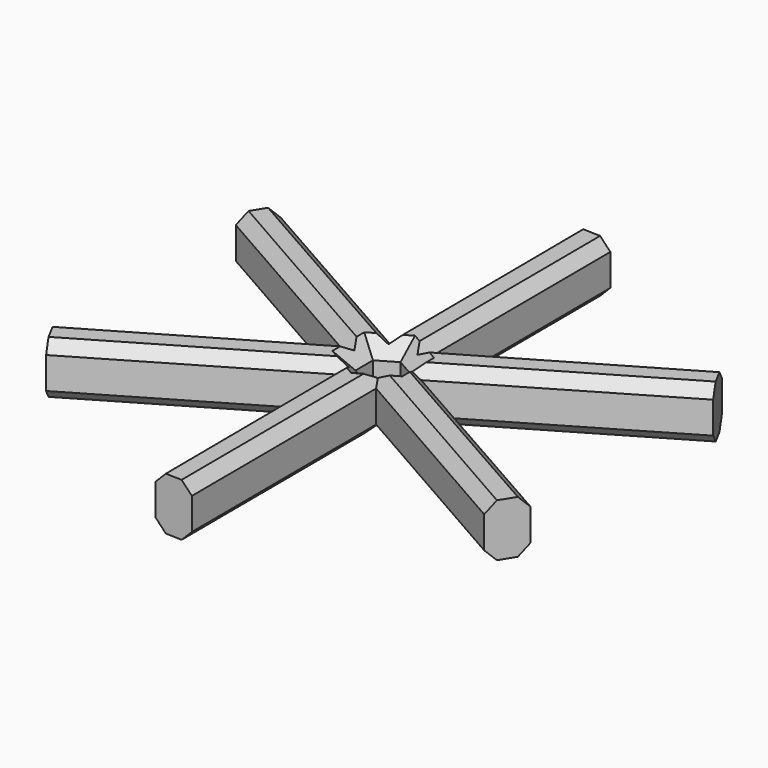
from build123d import *

# Parameters (mm, degrees)
F1_DEPTH      = 12.7
F2_SIZE       = 3.81
F3_T4_DEPTH   = 68.8298051047
F3_T9_DEPTH   = 68.1650882882
F3_T14_DEPTH  = 68.5414410237
F3_T19_DEPTH  = 68.5009740433
F3_T24_DEPTH  = 68.8298051047
F3_T29_DEPTH  = 68.1650882882
F3_T34_DEPTH  = 68.5414410237
F3_T39_DEPTH  = 68.5009740433
F3_T44_DEPTH  = 68.8298051047
F3_T49_DEPTH  = 68.1650882882
F3_T54_DEPTH  = 68.5414410237
F3_T59_DEPTH  = 68.5009740433
F3_T64_DEPTH  = 68.8298051047
F3_T69_DEPTH  = 68.1650882882
F3_T74_DEPTH  = 68.5414410237
F3_T79_DEPTH  = 68.5009740433
F3_T84_DEPTH  = 68.8298051047
F3_T89_DEPTH  = 68.1650882882
F3_T94_DEPTH  = 68.5414410237
F3_T99_DEPTH  = 68.5009740433
F3_T104_DEPTH = 68.8298051047
F3_T109_DEPTH = 68.1650882882
F3_T114_DEPTH = 68.5414410237
F3_T119_DEPTH = 68.5009740433
F3_T125_DEPTH = 68.8298051047
F3_T130_DEPTH = 68.1650882882
F3_T138_DEPTH = 68.5414410237
F3_T143_DEPTH = 68.5009740433
F3_T151_DEPTH = 68.8298051047
F3_T156_DEPTH = 68.1650882882
F3_T164_DEPTH = 68.5414410237
F3_T169_DEPTH = 68.5009740433
F3_T177_DEPTH = 68.8298051047
F3_T182_DEPTH = 68.1650882882
F3_T190_DEPTH = 68.5414410237
F3_T195_DEPTH = 68.5009740433
F3_T203_DEPTH = 68.8298051047
F3_T208_DEPTH = 68.1650882882
F3_T216_DEPTH = 68.5414410237
F3_T221_DEPTH = 68.5009740433
F3_T229_DEPTH = 68.8298051047
F3_T234_DEPTH = 68.1650882882
F3_T242_DEPTH = 68.5414410237
F3_T247_DEPTH = 68.5009740433
F3_T255_DEPTH = 68.8298051047
F3_T260_DEPTH = 68.1650882882
F3_T268_DEPTH = 68.5414410237
F3_T273_DEPTH = 68.5009740433


# Not quite as in the source:
# - a fillet or chamfer that OpenCascade refuses, or shapes differently, is made with other operations: its cross-section is extruded or revolved along the edge and cut away or added


with BuildPart() as f1:
    # F0 (on Top) → F1 (new body)
    with BuildSketch(Plane.XY):
        Polygon((4.2501981695, 63.0203421564), (-4.9943139693, 63.317529994), (-4.6016708631, 7.8416280415), (-0.0452432376, 5.2537971809), (4.5209166317, 7.9200684896), align=None)
        Polygon((-0.0452432376, 5.2537971809), (-4.6016708631, 7.8416280415), (-4.5646768909, 2.6148102364), align=None)
        Polygon((-4.5646768909, 2.6148102364), (-4.6016708631, 7.8416280415), (-52.8063450462, 35.2195551654), (-57.5503224335, 27.6004082668), (-9.1194388276, -0.0448055934), align=None)
        Polygon((-4.5273002062, -2.6660803836), (-4.5646768909, 2.6148102364), (-9.1194388276, -0.0448055934), align=None)
        Polygon((4.5209166317, 7.9200684896), (-0.0452432376, 5.2537971809), (4.5468305363, 2.6457210293), align=None)
        Polygon((52.6778159307, 36.03983709), (4.5209166317, 7.9200684896), (4.5468305363, 2.6457210293), (9.0918845225, 0.0643498466), (56.9042020064, 28.1218587083), align=None)
        Polygon((0.0178463546, -5.2605312658), (-4.5273002062, -2.6660803836), (-4.4902136594, -7.9059778881), align=None)
        Polygon((-4.4902136594, -7.9059778881), (-4.5273002062, -2.6660803836), (-9.1194388276, -0.0448055934), (-56.7023163474, -27.8293914923), (-52.3374324951, -35.9839677689), align=None)
        Polygon((9.0918845225, 0.0643498466), (4.5468305363, 2.6457210293), (4.5725434438, -2.5877167973), align=None)
        Polygon((0.0178463546, -5.2605312658), (-4.4902136594, -7.9059778881), (-4.0978569602, -63.3414138737), (4.8725065029, -63.6402453568), (4.5985221959, -7.8752628962), align=None)
        Polygon((4.5725434438, -2.5877167973), (0.0178463546, -5.2605312658), (4.5985221959, -7.8752628962), align=None)
        Polygon((9.0918845225, 0.0643498466), (4.5725434438, -2.5877167973), (4.5985221959, -7.8752628962), (52.4521181779, -35.1909506641), (57.3317464644, -27.3335622251), align=None)
    extrude(amount=F1_DEPTH)

    # F2
    f2_edges = [f1.edges().sort_by_distance(p)[0] for p in [
        (2.295195, -3.924124, 12.7),
        (-2.254727, -3.963306, 12.7),
        (-4.545989, -0.025635, 12.7),
        (-2.30496, 3.934304, 12.7),
        (2.250794, 3.949759, 12.7),
        (4.559687, 0.029002, 12.7),
        (-2.254727, -3.963306, 0),
        (2.295195, -3.924124, 0),
        (4.559687, 0.029002, 0),
        (2.250794, 3.949759, 0),
        (-2.30496, 3.934304, 0),
        (-4.545989, -0.025635, 0),
    ]]
    chamfer(f2_edges, length=F2_SIZE)

    # F3: chamfer of 2.54 on 24 edges, made by hand


with BuildPart() as f3_tool2:
    # F3_s3 → F3_t4 (new body)
    with BuildSketch(Plane(origin=(0.3448800676, -70.1946441039, 0), x_dir=(0, 0, 1), z_dir=(-0.004913137, 0.9999879305, 0))):
        Polygon((0, 2.0197744481), (2.54, 4.5597744481), (0, 4.5597744481), align=None)
    extrude(amount=F3_T4_DEPTH)

    split(bisect_by=Plane(origin=(-2.2604583159, -3.9600342448, 0), x_dir=(0, 0, 1), z_dir=(-0.4957390638, -0.8684715198, 0)), keep=Keep.TOP)


with BuildPart() as f1_1:
    add(f1.part)

    # F3_t1: cut F3_tool2
    add(f3_tool2.part, mode=Mode.SUBTRACT)


with BuildPart() as f3_tool7:
    # F3_s8 → F3_t9 (new body)
    with BuildSketch(Plane(origin=(1.186059592, -0.6770240109, 0), x_dir=(0, 0, 1), z_dir=(0.8684715198, -0.4957390638, 0))):
        Polygon((0, 2.0197744481), (2.54, 4.5597744481), (0, 4.5597744481), align=None)
    extrude(amount=F3_T9_DEPTH)

    split(bisect_by=Plane(origin=(4.5597194138, 0.0224027967, 0), x_dir=(0, 0, 1), z_dir=(0.9999879305, 0.004913137, 0)), keep=Keep.TOP)


with BuildPart() as f1_2:
    add(f1_1.part)

    # F3_t6: cut F3_tool7
    add(f3_tool7.part, mode=Mode.SUBTRACT)


with BuildPart() as f3_tool12:
    # F3_s13 → F3_t14 (new body)
    with BuildSketch(Plane(origin=(60.7665561884, -34.5124694876, 0), x_dir=(0, 0, 1), z_dir=(-0.8695424864, 0.4938581419, 0))):
        Polygon((0, 2.0060561225), (2.54, 4.5460561225), (0, 4.5460561225), align=None)
    extrude(amount=F3_T14_DEPTH)

    split(bisect_by=Plane(origin=(2.3008354316, -3.9208140208, 0), x_dir=(0, 0, 1), z_dir=(0.5061168119, -0.86246494, 0)), keep=Keep.TOP)


with BuildPart() as f1_3:
    add(f1_2.part)

    # F3_t11: cut F3_tool12
    add(f3_tool12.part, mode=Mode.SUBTRACT)


with BuildPart() as f3_tool17:
    # F3_s18 → F3_t19 (new body)
    with BuildSketch(Plane(origin=(1.1573635998, 0.6791709996, 0), x_dir=(0, 0, 1), z_dir=(0.86246494, 0.5061168119, 0))):
        Polygon((0, 2.0060561225), (2.54, 4.5460561225), (0, 4.5460561225), align=None)
    extrude(amount=F3_T19_DEPTH)

    split(bisect_by=Plane(origin=(2.2451068297, 3.952988944, 0), x_dir=(0, 0, 1), z_dir=(0.4938581419, 0.8695424864, 0)), keep=Keep.TOP)


with BuildPart() as f1_4:
    add(f1_3.part)

    # F3_t16: cut F3_tool17
    add(f3_tool17.part, mode=Mode.SUBTRACT)


with BuildPart() as f3_tool22:
    # F3_s23 → F3_t24 (new body)
    with BuildSketch(Plane(origin=(60.6179049697, 35.3959969517, 0), x_dir=(0, 0, 1), z_dir=(-0.8635583828, -0.5042488667, 0))):
        Polygon((0, 2.0197744481), (2.54, 4.5597744481), (0, 4.5597744481), align=None)
    extrude(amount=F3_T24_DEPTH)

    split(bisect_by=Plane(origin=(4.5597194138, 0.0224027967, 0), x_dir=(0, 0, 1), z_dir=(0.9999879305, 0.004913137, 0)), keep=Keep.TOP)


with BuildPart() as f1_5:
    add(f1_4.part)

    # F3_t21: cut F3_tool22
    add(f3_tool22.part, mode=Mode.SUBTRACT)


with BuildPart() as f3_tool27:
    # F3_s28 → F3_t29 (new body)
    with BuildSketch(Plane(origin=(-0.0067098036, 1.3656697426, 0), x_dir=(0, 0, 1), z_dir=(-0.004913137, 0.9999879305, 0))):
        Polygon((0, 2.0197744481), (2.54, 4.5597744481), (0, 4.5597744481), align=None)
    extrude(amount=F3_T29_DEPTH)

    split(bisect_by=Plane(origin=(-2.2992610979, 3.9376314481, 0), x_dir=(0, 0, 1), z_dir=(-0.5042488667, 0.8635583828, 0)), keep=Keep.TOP)


with BuildPart() as f1_6:
    add(f1_5.part)

    # F3_t26: cut F3_tool27
    add(f3_tool27.part, mode=Mode.SUBTRACT)


with BuildPart() as f3_tool32:
    # F3_s33 → F3_t34 (new body)
    with BuildSketch(Plane(origin=(-0.4946027707, 69.8816161035, 0), x_dir=(0, 0, 1), z_dir=(0.0070775464, -0.9999749539, 0))):
        Polygon((0, 2.0060561225), (2.54, 4.5460561225), (0, 4.5460561225), align=None)
    extrude(amount=F3_T34_DEPTH)

    split(bisect_by=Plane(origin=(2.2451068297, 3.952988944, 0), x_dir=(0, 0, 1), z_dir=(0.4938581419, 0.8695424864, 0)), keep=Keep.TOP)


with BuildPart() as f1_7:
    add(f1_6.part)

    # F3_t31: cut F3_tool32
    add(f3_tool32.part, mode=Mode.SUBTRACT)


with BuildPart() as f3_tool37:
    # F3_s38 → F3_t39 (new body)
    with BuildSketch(Plane(origin=(-1.1668611391, 0.6627207791, 0), x_dir=(0, 0, 1), z_dir=(-0.8695424864, 0.4938581419, 0))):
        Polygon((0, 2.0060561225), (2.54, 4.5460561225), (0, 4.5460561225), align=None)
    extrude(amount=F3_T39_DEPTH)

    split(bisect_by=Plane(origin=(-4.5459422613, -0.0321749233, 0), x_dir=(0, 0, 1), z_dir=(-0.9999749539, -0.0070775464, 0)), keep=Keep.TOP)


with BuildPart() as f1_8:
    add(f1_7.part)

    # F3_t36: cut F3_tool37
    add(f3_tool37.part, mode=Mode.SUBTRACT)


with BuildPart() as f3_tool42:
    # F3_s43 → F3_t44 (new body)
    with BuildSketch(Plane(origin=(-60.9627850374, 34.7986471521, 0), x_dir=(0, 0, 1), z_dir=(0.8684715198, -0.4957390638, 0))):
        Polygon((0, 2.0197744481), (2.54, 4.5597744481), (0, 4.5597744481), align=None)
    extrude(amount=F3_T44_DEPTH)

    split(bisect_by=Plane(origin=(-2.2992610979, 3.9376314481, 0), x_dir=(0, 0, 1), z_dir=(-0.5042488667, 0.8635583828, 0)), keep=Keep.TOP)


with BuildPart() as f1_9:
    add(f1_8.part)

    # F3_t41: cut F3_tool42
    add(f3_tool42.part, mode=Mode.SUBTRACT)


with BuildPart() as f3_tool47:
    # F3_s48 → F3_t49 (new body)
    with BuildSketch(Plane(origin=(-1.1793497885, -0.6886457316, 0), x_dir=(0, 0, 1), z_dir=(-0.8635583828, -0.5042488667, 0))):
        Polygon((0, 2.0197744481), (2.54, 4.5597744481), (0, 4.5597744481), align=None)
    extrude(amount=F3_T49_DEPTH)

    split(bisect_by=Plane(origin=(-2.2604583159, -3.9600342448, 0), x_dir=(0, 0, 1), z_dir=(-0.4957390638, -0.8684715198, 0)), keep=Keep.TOP)


with BuildPart() as f1_10:
    add(f1_9.part)

    # F3_t46: cut F3_tool47
    add(f3_tool47.part, mode=Mode.SUBTRACT)


with BuildPart() as f3_tool52:
    # F3_s53 → F3_t54 (new body)
    with BuildSketch(Plane(origin=(-60.2719534178, -35.3691466159, 0), x_dir=(0, 0, 1), z_dir=(0.86246494, 0.5061168119, 0))):
        Polygon((0, 2.0060561225), (2.54, 4.5460561225), (0, 4.5460561225), align=None)
    extrude(amount=F3_T54_DEPTH)

    split(bisect_by=Plane(origin=(-4.5459422613, -0.0321749233, 0), x_dir=(0, 0, 1), z_dir=(-0.9999749539, -0.0070775464, 0)), keep=Keep.TOP)


with BuildPart() as f1_11:
    add(f1_10.part)

    # F3_t51: cut F3_tool52
    add(f3_tool52.part, mode=Mode.SUBTRACT)


with BuildPart() as f3_tool57:
    # F3_s58 → F3_t59 (new body)
    with BuildSketch(Plane(origin=(0.0094975392, -1.3418917787, 0), x_dir=(0, 0, 1), z_dir=(0.0070775464, -0.9999749539, 0))):
        Polygon((0, 2.0060561225), (2.54, 4.5460561225), (0, 4.5460561225), align=None)
    extrude(amount=F3_T59_DEPTH)

    split(bisect_by=Plane(origin=(2.3008354316, -3.9208140208, 0), x_dir=(0, 0, 1), z_dir=(0.5061168119, -0.86246494, 0)), keep=Keep.TOP)


with BuildPart() as f1_12:
    add(f1_11.part)

    # F3_t56: cut F3_tool57
    add(f3_tool57.part, mode=Mode.SUBTRACT)


with BuildPart() as f3_tool62:
    # F3_s63 → F3_t64 (new body)
    with BuildSketch(Plane(origin=(0.3448800676, -70.1946441039, 0), x_dir=(0, 0, 1), z_dir=(-0.004913137, 0.9999879305, 0))):
        Polygon((12.7, 2.0197744481), (10.16, 4.5597744481), (12.7, 4.5597744481), align=None)
    extrude(amount=F3_T64_DEPTH)

    split(bisect_by=Plane(origin=(-2.2604583159, -3.9600342448, 0), x_dir=(0, 0, 1), z_dir=(-0.4957390638, -0.8684715198, 0)), keep=Keep.TOP)


with BuildPart() as f1_13:
    add(f1_12.part)

    # F3_t61: cut F3_tool62
    add(f3_tool62.part, mode=Mode.SUBTRACT)


with BuildPart() as f3_tool67:
    # F3_s68 → F3_t69 (new body)
    with BuildSketch(Plane(origin=(1.186059592, -0.6770240109, 0), x_dir=(0, 0, 1), z_dir=(0.8684715198, -0.4957390638, 0))):
        Polygon((12.7, 2.0197744481), (10.16, 4.5597744481), (12.7, 4.5597744481), align=None)
    extrude(amount=F3_T69_DEPTH)

    split(bisect_by=Plane(origin=(4.5597194138, 0.0224027967, 0), x_dir=(0, 0, 1), z_dir=(0.9999879305, 0.004913137, 0)), keep=Keep.TOP)


with BuildPart() as f1_14:
    add(f1_13.part)

    # F3_t66: cut F3_tool67
    add(f3_tool67.part, mode=Mode.SUBTRACT)


with BuildPart() as f3_tool72:
    # F3_s73 → F3_t74 (new body)
    with BuildSketch(Plane(origin=(60.7665561884, -34.5124694876, 0), x_dir=(0, 0, 1), z_dir=(-0.8695424864, 0.4938581419, 0))):
        Polygon((12.7, 2.0060561225), (10.16, 4.5460561225), (12.7, 4.5460561225), align=None)
    extrude(amount=F3_T74_DEPTH)

    split(bisect_by=Plane(origin=(2.3008354316, -3.9208140208, 0), x_dir=(0, 0, 1), z_dir=(0.5061168119, -0.86246494, 0)), keep=Keep.TOP)


with BuildPart() as f1_15:
    add(f1_14.part)

    # F3_t71: cut F3_tool72
    add(f3_tool72.part, mode=Mode.SUBTRACT)


with BuildPart() as f3_tool77:
    # F3_s78 → F3_t79 (new body)
    with BuildSketch(Plane(origin=(1.1573635998, 0.6791709996, 0), x_dir=(0, 0, 1), z_dir=(0.86246494, 0.5061168119, 0))):
        Polygon((12.7, 2.0060561225), (10.16, 4.5460561225), (12.7, 4.5460561225), align=None)
    extrude(amount=F3_T79_DEPTH)

    split(bisect_by=Plane(origin=(2.2451068297, 3.952988944, 0), x_dir=(0, 0, 1), z_dir=(0.4938581419, 0.8695424864, 0)), keep=Keep.TOP)


with BuildPart() as f1_16:
    add(f1_15.part)

    # F3_t76: cut F3_tool77
    add(f3_tool77.part, mode=Mode.SUBTRACT)


with BuildPart() as f3_tool82:
    # F3_s83 → F3_t84 (new body)
    with BuildSketch(Plane(origin=(60.6179049697, 35.3959969517, 0), x_dir=(0, 0, 1), z_dir=(-0.8635583828, -0.5042488667, 0))):
        Polygon((12.7, 2.0197744481), (10.16, 4.5597744481), (12.7, 4.5597744481), align=None)
    extrude(amount=F3_T84_DEPTH)

    split(bisect_by=Plane(origin=(4.5597194138, 0.0224027967, 0), x_dir=(0, 0, 1), z_dir=(0.9999879305, 0.004913137, 0)), keep=Keep.TOP)


with BuildPart() as f1_17:
    add(f1_16.part)

    # F3_t81: cut F3_tool82
    add(f3_tool82.part, mode=Mode.SUBTRACT)


with BuildPart() as f3_tool87:
    # F3_s88 → F3_t89 (new body)
    with BuildSketch(Plane(origin=(-0.0067098036, 1.3656697426, 0), x_dir=(0, 0, 1), z_dir=(-0.004913137, 0.9999879305, 0))):
        Polygon((12.7, 2.0197744481), (10.16, 4.5597744481), (12.7, 4.5597744481), align=None)
    extrude(amount=F3_T89_DEPTH)

    split(bisect_by=Plane(origin=(-2.2992610979, 3.9376314481, 0), x_dir=(0, 0, 1), z_dir=(-0.5042488667, 0.8635583828, 0)), keep=Keep.TOP)


with BuildPart() as f1_18:
    add(f1_17.part)

    # F3_t86: cut F3_tool87
    add(f3_tool87.part, mode=Mode.SUBTRACT)


with BuildPart() as f3_tool92:
    # F3_s93 → F3_t94 (new body)
    with BuildSketch(Plane(origin=(-0.4946027707, 69.8816161035, 0), x_dir=(0, 0, 1), z_dir=(0.0070775464, -0.9999749539, 0))):
        Polygon((12.7, 2.0060561225), (10.16, 4.5460561225), (12.7, 4.5460561225), align=None)
    extrude(amount=F3_T94_DEPTH)

    split(bisect_by=Plane(origin=(2.2451068297, 3.952988944, 0), x_dir=(0, 0, 1), z_dir=(0.4938581419, 0.8695424864, 0)), keep=Keep.TOP)


with BuildPart() as f1_19:
    add(f1_18.part)

    # F3_t91: cut F3_tool92
    add(f3_tool92.part, mode=Mode.SUBTRACT)


with BuildPart() as f3_tool97:
    # F3_s98 → F3_t99 (new body)
    with BuildSketch(Plane(origin=(-1.1668611391, 0.6627207791, 0), x_dir=(0, 0, 1), z_dir=(-0.8695424864, 0.4938581419, 0))):
        Polygon((12.7, 2.0060561225), (10.16, 4.5460561225), (12.7, 4.5460561225), align=None)
    extrude(amount=F3_T99_DEPTH)

    split(bisect_by=Plane(origin=(-4.5459422613, -0.0321749233, 0), x_dir=(0, 0, 1), z_dir=(-0.9999749539, -0.0070775464, 0)), keep=Keep.TOP)


with BuildPart() as f1_20:
    add(f1_19.part)

    # F3_t96: cut F3_tool97
    add(f3_tool97.part, mode=Mode.SUBTRACT)


with BuildPart() as f3_tool102:
    # F3_s103 → F3_t104 (new body)
    with BuildSketch(Plane(origin=(-60.9627850374, 34.7986471521, 0), x_dir=(0, 0, 1), z_dir=(0.8684715198, -0.4957390638, 0))):
        Polygon((12.7, 2.0197744481), (10.16, 4.5597744481), (12.7, 4.5597744481), align=None)
    extrude(amount=F3_T104_DEPTH)

    split(bisect_by=Plane(origin=(-2.2992610979, 3.9376314481, 0), x_dir=(0, 0, 1), z_dir=(-0.5042488667, 0.8635583828, 0)), keep=Keep.TOP)


with BuildPart() as f1_21:
    add(f1_20.part)

    # F3_t101: cut F3_tool102
    add(f3_tool102.part, mode=Mode.SUBTRACT)


with BuildPart() as f3_tool107:
    # F3_s108 → F3_t109 (new body)
    with BuildSketch(Plane(origin=(-1.1793497885, -0.6886457316, 0), x_dir=(0, 0, 1), z_dir=(-0.8635583828, -0.5042488667, 0))):
        Polygon((12.7, 2.0197744481), (10.16, 4.5597744481), (12.7, 4.5597744481), align=None)
    extrude(amount=F3_T109_DEPTH)

    split(bisect_by=Plane(origin=(-2.2604583159, -3.9600342448, 0), x_dir=(0, 0, 1), z_dir=(-0.4957390638, -0.8684715198, 0)), keep=Keep.TOP)


with BuildPart() as f1_22:
    add(f1_21.part)

    # F3_t106: cut F3_tool107
    add(f3_tool107.part, mode=Mode.SUBTRACT)


with BuildPart() as f3_tool112:
    # F3_s113 → F3_t114 (new body)
    with BuildSketch(Plane(origin=(-60.2719534178, -35.3691466159, 0), x_dir=(0, 0, 1), z_dir=(0.86246494, 0.5061168119, 0))):
        Polygon((12.7, 2.0060561225), (10.16, 4.5460561225), (12.7, 4.5460561225), align=None)
    extrude(amount=F3_T114_DEPTH)

    split(bisect_by=Plane(origin=(-4.5459422613, -0.0321749233, 0), x_dir=(0, 0, 1), z_dir=(-0.9999749539, -0.0070775464, 0)), keep=Keep.TOP)


with BuildPart() as f1_23:
    add(f1_22.part)

    # F3_t111: cut F3_tool112
    add(f3_tool112.part, mode=Mode.SUBTRACT)


with BuildPart() as f3_tool117:
    # F3_s118 → F3_t119 (new body)
    with BuildSketch(Plane(origin=(0.0094975392, -1.3418917787, 0), x_dir=(0, 0, 1), z_dir=(0.0070775464, -0.9999749539, 0))):
        Polygon((12.7, 2.0060561225), (10.16, 4.5460561225), (12.7, 4.5460561225), align=None)
    extrude(amount=F3_T119_DEPTH)

    split(bisect_by=Plane(origin=(2.3008354316, -3.9208140208, 0), x_dir=(0, 0, 1), z_dir=(0.5061168119, -0.86246494, 0)), keep=Keep.TOP)


with BuildPart() as f1_24:
    add(f1_23.part)

    # F3_t116: cut F3_tool117
    add(f3_tool117.part, mode=Mode.SUBTRACT)


with BuildPart() as f3_tool123:
    # F3_s124 → F3_t125 (new body)
    with BuildSketch(Plane(origin=(0.3448800676, -70.1946441039, 0), x_dir=(0, 0, 1), z_dir=(-0.004913137, 0.9999879305, 0))):
        Polygon((0, 2.0197744481), (2.54, 4.5597744481), (0, 4.5597744481), align=None)
    extrude(amount=F3_T125_DEPTH)

    split(bisect_by=Plane(origin=(2.1145702425, -3.603402721, 4.1780280612), x_dir=(0.86246494, 0.5061168119, 0), z_dir=(0.3578786298, -0.6098548076, 0.7071067812)), keep=Keep.TOP)

    split(bisect_by=Plane(origin=(-2.2604583159, -3.9600342448, 0), x_dir=(0, 0, 1), z_dir=(0.4957390638, 0.8684715198, 0)), keep=Keep.TOP)


with BuildPart() as f3_tool128:
    # F3_s129 → F3_t130 (new body)
    with BuildSketch(Plane(origin=(1.186059592, -0.6770240109, 0), x_dir=(0, 0, 1), z_dir=(0.8684715198, -0.4957390638, 0))):
        Polygon((0, 2.0197744481), (2.54, 4.5597744481), (0, 4.5597744481), align=None)
    extrude(amount=F3_T130_DEPTH)

    split(bisect_by=Plane(origin=(2.1145702425, -3.603402721, 4.1780280612), x_dir=(0.86246494, 0.5061168119, 0), z_dir=(0.3578786298, -0.6098548076, 0.7071067812)), keep=Keep.TOP)

    split(bisect_by=Plane(origin=(4.5597194138, 0.0224027967, 0), x_dir=(0, 0, 1), z_dir=(-0.9999879305, -0.004913137, 0)), keep=Keep.TOP)


with BuildPart() as f3_tool123_1:
    add(f3_tool123.part)

    # F3_t133: intersect F3_tool128
    add(f3_tool128.part, mode=Mode.INTERSECT)


with BuildPart() as f1_25:
    add(f1_24.part)

    # F3_t121: cut F3_tool123
    add(f3_tool123_1.part, mode=Mode.SUBTRACT)


with BuildPart() as f3_tool136:
    # F3_s137 → F3_t138 (new body)
    with BuildSketch(Plane(origin=(60.7665561884, -34.5124694876, 0), x_dir=(0, 0, 1), z_dir=(-0.8695424864, 0.4938581419, 0))):
        Polygon((0, 2.0060561225), (2.54, 4.5460561225), (0, 4.5460561225), align=None)
    extrude(amount=F3_T138_DEPTH)

    split(bisect_by=Plane(origin=(4.1848367144, 0.0205609244, 4.1848872241), x_dir=(-0.004913137, 0.9999879305, 0), z_dir=(0.7070982467, 0.0034741125, 0.7071067812)), keep=Keep.TOP)

    split(bisect_by=Plane(origin=(2.3008354316, -3.9208140208, 0), x_dir=(0, 0, 1), z_dir=(-0.5061168119, 0.86246494, 0)), keep=Keep.TOP)


with BuildPart() as f3_tool141:
    # F3_s142 → F3_t143 (new body)
    with BuildSketch(Plane(origin=(1.1573635998, 0.6791709996, 0), x_dir=(0, 0, 1), z_dir=(0.86246494, 0.5061168119, 0))):
        Polygon((0, 2.0060561225), (2.54, 4.5460561225), (0, 4.5460561225), align=None)
    extrude(amount=F3_T143_DEPTH)

    split(bisect_by=Plane(origin=(4.1848367144, 0.0205609244, 4.1848872241), x_dir=(-0.004913137, 0.9999879305, 0), z_dir=(0.7070982467, 0.0034741125, 0.7071067812)), keep=Keep.TOP)

    split(bisect_by=Plane(origin=(2.2451068297, 3.952988944, 0), x_dir=(0, 0, 1), z_dir=(-0.4938581419, -0.8695424864, 0)), keep=Keep.TOP)


with BuildPart() as f3_tool136_1:
    add(f3_tool136.part)

    # F3_t146: intersect F3_tool141
    add(f3_tool141.part, mode=Mode.INTERSECT)


with BuildPart() as f1_26:
    add(f1_25.part)

    # F3_t134: cut F3_tool136
    add(f3_tool136_1.part, mode=Mode.SUBTRACT)


with BuildPart() as f3_tool149:
    # F3_s150 → F3_t151 (new body)
    with BuildSketch(Plane(origin=(60.6179049697, 35.3959969517, 0), x_dir=(0, 0, 1), z_dir=(-0.8635583828, -0.5042488667, 0))):
        Polygon((0, 2.0197744481), (2.54, 4.5597744481), (0, 4.5597744481), align=None)
    extrude(amount=F3_T151_DEPTH)

    split(bisect_by=Plane(origin=(2.0633531752, 3.6329729086, 4.1780280612), x_dir=(-0.8695424864, 0.4938581419, 0), z_dir=(0.3492104411, 0.6148593887, 0.7071067812)), keep=Keep.TOP)

    split(bisect_by=Plane(origin=(4.5597194138, 0.0224027967, 0), x_dir=(0, 0, 1), z_dir=(-0.9999879305, -0.004913137, 0)), keep=Keep.TOP)


with BuildPart() as f3_tool154:
    # F3_s155 → F3_t156 (new body)
    with BuildSketch(Plane(origin=(-0.0067098036, 1.3656697426, 0), x_dir=(0, 0, 1), z_dir=(-0.004913137, 0.9999879305, 0))):
        Polygon((0, 2.0197744481), (2.54, 4.5597744481), (0, 4.5597744481), align=None)
    extrude(amount=F3_T156_DEPTH)

    split(bisect_by=Plane(origin=(2.0633531752, 3.6329729086, 4.1780280612), x_dir=(-0.8695424864, 0.4938581419, 0), z_dir=(0.3492104411, 0.6148593887, 0.7071067812)), keep=Keep.TOP)

    split(bisect_by=Plane(origin=(-2.2992610979, 3.9376314481, 0), x_dir=(0, 0, 1), z_dir=(0.5042488667, -0.8635583828, 0)), keep=Keep.TOP)


with BuildPart() as f3_tool149_1:
    add(f3_tool149.part)

    # F3_t159: intersect F3_tool154
    add(f3_tool154.part, mode=Mode.INTERSECT)


with BuildPart() as f1_27:
    add(f1_26.part)

    # F3_t147: cut F3_tool149
    add(f3_tool149_1.part, mode=Mode.SUBTRACT)


with BuildPart() as f3_tool162:
    # F3_s163 → F3_t164 (new body)
    with BuildSketch(Plane(origin=(-0.4946027707, 69.8816161035, 0), x_dir=(0, 0, 1), z_dir=(0.0070775464, -0.9999749539, 0))):
        Polygon((0, 2.0060561225), (2.54, 4.5460561225), (0, 4.5460561225), align=None)
    extrude(amount=F3_T164_DEPTH)

    split(bisect_by=Plane(origin=(-2.1102246401, 3.6138944432, 4.1848872241), x_dir=(-0.8635583828, -0.5042488667, 0), z_dir=(-0.3565577931, 0.6106279884, 0.7071067812)), keep=Keep.TOP)

    split(bisect_by=Plane(origin=(2.2451068297, 3.952988944, 0), x_dir=(0, 0, 1), z_dir=(-0.4938581419, -0.8695424864, 0)), keep=Keep.TOP)


with BuildPart() as f3_tool167:
    # F3_s168 → F3_t169 (new body)
    with BuildSketch(Plane(origin=(-1.1668611391, 0.6627207791, 0), x_dir=(0, 0, 1), z_dir=(-0.8695424864, 0.4938581419, 0))):
        Polygon((0, 2.0060561225), (2.54, 4.5460561225), (0, 4.5460561225), align=None)
    extrude(amount=F3_T169_DEPTH)

    split(bisect_by=Plane(origin=(-2.1102246401, 3.6138944432, 4.1848872241), x_dir=(-0.8635583828, -0.5042488667, 0), z_dir=(-0.3565577931, 0.6106279884, 0.7071067812)), keep=Keep.TOP)

    split(bisect_by=Plane(origin=(-4.5459422613, -0.0321749233, 0), x_dir=(0, 0, 1), z_dir=(0.9999749539, 0.0070775464, 0)), keep=Keep.TOP)


with BuildPart() as f3_tool162_1:
    add(f3_tool162.part)

    # F3_t172: intersect F3_tool167
    add(f3_tool167.part, mode=Mode.INTERSECT)


with BuildPart() as f1_28:
    add(f1_27.part)

    # F3_t160: cut F3_tool162
    add(f3_tool162_1.part, mode=Mode.SUBTRACT)


with BuildPart() as f3_tool175:
    # F3_s176 → F3_t177 (new body)
    with BuildSketch(Plane(origin=(-60.9627850374, 34.7986471521, 0), x_dir=(0, 0, 1), z_dir=(0.8684715198, -0.4957390638, 0))):
        Polygon((0, 2.0197744481), (2.54, 4.5597744481), (0, 4.5597744481), align=None)
    extrude(amount=F3_T177_DEPTH)

    split(bisect_by=Plane(origin=(-4.1779234177, -0.0295701876, 4.1780280612), x_dir=(0.0070775464, -0.9999749539, 0), z_dir=(-0.7070890709, -0.0050045811, 0.7071067812)), keep=Keep.TOP)

    split(bisect_by=Plane(origin=(-2.2992610979, 3.9376314481, 0), x_dir=(0, 0, 1), z_dir=(0.5042488667, -0.8635583828, 0)), keep=Keep.TOP)


with BuildPart() as f3_tool180:
    # F3_s181 → F3_t182 (new body)
    with BuildSketch(Plane(origin=(-1.1793497885, -0.6886457316, 0), x_dir=(0, 0, 1), z_dir=(-0.8635583828, -0.5042488667, 0))):
        Polygon((0, 2.0197744481), (2.54, 4.5597744481), (0, 4.5597744481), align=None)
    extrude(amount=F3_T182_DEPTH)

    split(bisect_by=Plane(origin=(-4.1779234177, -0.0295701876, 4.1780280612), x_dir=(0.0070775464, -0.9999749539, 0), z_dir=(-0.7070890709, -0.0050045811, 0.7071067812)), keep=Keep.TOP)

    split(bisect_by=Plane(origin=(-2.2604583159, -3.9600342448, 0), x_dir=(0, 0, 1), z_dir=(0.4957390638, 0.8684715198, 0)), keep=Keep.TOP)


with BuildPart() as f3_tool175_1:
    add(f3_tool175.part)

    # F3_t185: intersect F3_tool180
    add(f3_tool180.part, mode=Mode.INTERSECT)


with BuildPart() as f1_29:
    add(f1_28.part)

    # F3_t173: cut F3_tool175
    add(f3_tool175_1.part, mode=Mode.SUBTRACT)


with BuildPart() as f3_tool188:
    # F3_s189 → F3_t190 (new body)
    with BuildSketch(Plane(origin=(-60.2719534178, -35.3691466159, 0), x_dir=(0, 0, 1), z_dir=(0.86246494, 0.5061168119, 0))):
        Polygon((0, 2.0060561225), (2.54, 4.5460561225), (0, 4.5460561225), align=None)
    extrude(amount=F3_T190_DEPTH)

    split(bisect_by=Plane(origin=(-2.0746120744, -3.6344553676, 4.1848872241), x_dir=(0.8684715198, -0.4957390638, 0), z_dir=(-0.3505404537, -0.6141021009, 0.7071067812)), keep=Keep.TOP)

    split(bisect_by=Plane(origin=(-4.5459422613, -0.0321749233, 0), x_dir=(0, 0, 1), z_dir=(0.9999749539, 0.0070775464, 0)), keep=Keep.TOP)


with BuildPart() as f3_tool193:
    # F3_s194 → F3_t195 (new body)
    with BuildSketch(Plane(origin=(0.0094975392, -1.3418917787, 0), x_dir=(0, 0, 1), z_dir=(0.0070775464, -0.9999749539, 0))):
        Polygon((0, 2.0060561225), (2.54, 4.5460561225), (0, 4.5460561225), align=None)
    extrude(amount=F3_T195_DEPTH)

    split(bisect_by=Plane(origin=(-2.0746120744, -3.6344553676, 4.1848872241), x_dir=(0.8684715198, -0.4957390638, 0), z_dir=(-0.3505404537, -0.6141021009, 0.7071067812)), keep=Keep.TOP)

    split(bisect_by=Plane(origin=(2.3008354316, -3.9208140208, 0), x_dir=(0, 0, 1), z_dir=(-0.5061168119, 0.86246494, 0)), keep=Keep.TOP)


with BuildPart() as f3_tool188_1:
    add(f3_tool188.part)

    # F3_t198: intersect F3_tool193
    add(f3_tool193.part, mode=Mode.INTERSECT)


with BuildPart() as f1_30:
    add(f1_29.part)

    # F3_t186: cut F3_tool188
    add(f3_tool188_1.part, mode=Mode.SUBTRACT)


with BuildPart() as f3_tool201:
    # F3_s202 → F3_t203 (new body)
    with BuildSketch(Plane(origin=(0.3448800676, -70.1946441039, 0), x_dir=(0, 0, 1), z_dir=(-0.004913137, 0.9999879305, 0))):
        Polygon((12.7, 2.0197744481), (10.16, 4.5597744481), (12.7, 4.5597744481), align=None)
    extrude(amount=F3_T203_DEPTH)

    split(bisect_by=Plane(origin=(-1.0992715133, 1.8732496478, 2.1719719388), x_dir=(0.86246494, 0.5061168119, 0), z_dir=(0.3578786298, -0.6098548076, -0.7071067812)), keep=Keep.TOP)

    split(bisect_by=Plane(origin=(-2.2604583159, -3.9600342448, 0), x_dir=(0, 0, 1), z_dir=(0.4957390638, 0.8684715198, 0)), keep=Keep.TOP)


with BuildPart() as f3_tool206:
    # F3_s207 → F3_t208 (new body)
    with BuildSketch(Plane(origin=(1.186059592, -0.6770240109, 0), x_dir=(0, 0, 1), z_dir=(0.8684715198, -0.4957390638, 0))):
        Polygon((12.7, 2.0197744481), (10.16, 4.5597744481), (12.7, 4.5597744481), align=None)
    extrude(amount=F3_T208_DEPTH)

    split(bisect_by=Plane(origin=(-1.0992715133, 1.8732496478, 2.1719719388), x_dir=(0.86246494, 0.5061168119, 0), z_dir=(0.3578786298, -0.6098548076, -0.7071067812)), keep=Keep.TOP)

    split(bisect_by=Plane(origin=(4.5597194138, 0.0224027967, 0), x_dir=(0, 0, 1), z_dir=(-0.9999879305, -0.004913137, 0)), keep=Keep.TOP)


with BuildPart() as f3_tool201_1:
    add(f3_tool201.part)

    # F3_t211: intersect F3_tool206
    add(f3_tool206.part, mode=Mode.INTERSECT)


with BuildPart() as f1_31:
    add(f1_30.part)

    # F3_t199: cut F3_tool201
    add(f3_tool201_1.part, mode=Mode.SUBTRACT)


with BuildPart() as f3_tool214:
    # F3_s215 → F3_t216 (new body)
    with BuildSketch(Plane(origin=(60.7665561884, -34.5124694876, 0), x_dir=(0, 0, 1), z_dir=(-0.8695424864, 0.4938581419, 0))):
        Polygon((12.7, 2.0060561225), (10.16, 4.5460561225), (12.7, 4.5460561225), align=None)
    extrude(amount=F3_T216_DEPTH)

    split(bisect_by=Plane(origin=(-2.165086644, -0.0106374957, 2.1651127759), x_dir=(-0.004913137, 0.9999879305, 0), z_dir=(0.7070982467, 0.0034741125, -0.7071067812)), keep=Keep.TOP)

    split(bisect_by=Plane(origin=(2.3008354316, -3.9208140208, 0), x_dir=(0, 0, 1), z_dir=(-0.5061168119, 0.86246494, 0)), keep=Keep.TOP)


with BuildPart() as f3_tool219:
    # F3_s220 → F3_t221 (new body)
    with BuildSketch(Plane(origin=(1.1573635998, 0.6791709996, 0), x_dir=(0, 0, 1), z_dir=(0.86246494, 0.5061168119, 0))):
        Polygon((12.7, 2.0060561225), (10.16, 4.5460561225), (12.7, 4.5460561225), align=None)
    extrude(amount=F3_T221_DEPTH)

    split(bisect_by=Plane(origin=(-2.165086644, -0.0106374957, 2.1651127759), x_dir=(-0.004913137, 0.9999879305, 0), z_dir=(0.7070982467, 0.0034741125, -0.7071067812)), keep=Keep.TOP)

    split(bisect_by=Plane(origin=(2.2451068297, 3.952988944, 0), x_dir=(0, 0, 1), z_dir=(-0.4938581419, -0.8695424864, 0)), keep=Keep.TOP)


with BuildPart() as f3_tool214_1:
    add(f3_tool214.part)

    # F3_t224: intersect F3_tool219
    add(f3_tool219.part, mode=Mode.INTERSECT)


with BuildPart() as f1_32:
    add(f1_31.part)

    # F3_t212: cut F3_tool214
    add(f3_tool214_1.part, mode=Mode.SUBTRACT)


with BuildPart() as f3_tool227:
    # F3_s228 → F3_t229 (new body)
    with BuildSketch(Plane(origin=(60.6179049697, 35.3959969517, 0), x_dir=(0, 0, 1), z_dir=(-0.8635583828, -0.5042488667, 0))):
        Polygon((12.7, 2.0197744481), (10.16, 4.5597744481), (12.7, 4.5597744481), align=None)
    extrude(amount=F3_T229_DEPTH)

    split(bisect_by=Plane(origin=(-1.072646026, -1.88862188, 2.1719719388), x_dir=(-0.8695424864, 0.4938581419, 0), z_dir=(0.3492104411, 0.6148593887, -0.7071067812)), keep=Keep.TOP)

    split(bisect_by=Plane(origin=(4.5597194138, 0.0224027967, 0), x_dir=(0, 0, 1), z_dir=(-0.9999879305, -0.004913137, 0)), keep=Keep.TOP)


with BuildPart() as f3_tool232:
    # F3_s233 → F3_t234 (new body)
    with BuildSketch(Plane(origin=(-0.0067098036, 1.3656697426, 0), x_dir=(0, 0, 1), z_dir=(-0.004913137, 0.9999879305, 0))):
        Polygon((12.7, 2.0197744481), (10.16, 4.5597744481), (12.7, 4.5597744481), align=None)
    extrude(amount=F3_T234_DEPTH)

    split(bisect_by=Plane(origin=(-1.072646026, -1.88862188, 2.1719719388), x_dir=(-0.8695424864, 0.4938581419, 0), z_dir=(0.3492104411, 0.6148593887, -0.7071067812)), keep=Keep.TOP)

    split(bisect_by=Plane(origin=(-2.2992610979, 3.9376314481, 0), x_dir=(0, 0, 1), z_dir=(0.5042488667, -0.8635583828, 0)), keep=Keep.TOP)


with BuildPart() as f3_tool227_1:
    add(f3_tool227.part)

    # F3_t237: intersect F3_tool232
    add(f3_tool232.part, mode=Mode.INTERSECT)


with BuildPart() as f1_33:
    add(f1_32.part)

    # F3_t225: cut F3_tool227
    add(f3_tool227_1.part, mode=Mode.SUBTRACT)


with BuildPart() as f3_tool240:
    # F3_s241 → F3_t242 (new body)
    with BuildSketch(Plane(origin=(-0.4946027707, 69.8816161035, 0), x_dir=(0, 0, 1), z_dir=(0.0070775464, -0.9999749539, 0))):
        Polygon((12.7, 2.0060561225), (10.16, 4.5460561225), (12.7, 4.5460561225), align=None)
    extrude(amount=F3_T242_DEPTH)

    split(bisect_by=Plane(origin=(1.0917556636, -1.8697012873, 2.1651127759), x_dir=(-0.8635583828, -0.5042488667, 0), z_dir=(-0.3565577931, 0.6106279884, -0.7071067812)), keep=Keep.TOP)

    split(bisect_by=Plane(origin=(2.2451068297, 3.952988944, 0), x_dir=(0, 0, 1), z_dir=(-0.4938581419, -0.8695424864, 0)), keep=Keep.TOP)


with BuildPart() as f3_tool245:
    # F3_s246 → F3_t247 (new body)
    with BuildSketch(Plane(origin=(-1.1668611391, 0.6627207791, 0), x_dir=(0, 0, 1), z_dir=(-0.8695424864, 0.4938581419, 0))):
        Polygon((12.7, 2.0060561225), (10.16, 4.5460561225), (12.7, 4.5460561225), align=None)
    extrude(amount=F3_T247_DEPTH)

    split(bisect_by=Plane(origin=(1.0917556636, -1.8697012873, 2.1651127759), x_dir=(-0.8635583828, -0.5042488667, 0), z_dir=(-0.3565577931, 0.6106279884, -0.7071067812)), keep=Keep.TOP)

    split(bisect_by=Plane(origin=(-4.5459422613, -0.0321749233, 0), x_dir=(0, 0, 1), z_dir=(0.9999749539, 0.0070775464, 0)), keep=Keep.TOP)


with BuildPart() as f3_tool240_1:
    add(f3_tool240.part)

    # F3_t250: intersect F3_tool245
    add(f3_tool245.part, mode=Mode.INTERSECT)


with BuildPart() as f1_34:
    add(f1_33.part)

    # F3_t238: cut F3_tool240
    add(f3_tool240_1.part, mode=Mode.SUBTRACT)


with BuildPart() as f3_tool253:
    # F3_s254 → F3_t255 (new body)
    with BuildSketch(Plane(origin=(-60.9627850374, 34.7986471521, 0), x_dir=(0, 0, 1), z_dir=(0.8684715198, -0.4957390638, 0))):
        Polygon((12.7, 2.0197744481), (10.16, 4.5597744481), (12.7, 4.5597744481), align=None)
    extrude(amount=F3_T255_DEPTH)

    split(bisect_by=Plane(origin=(-2.2992610979, 3.9376314481, 0), x_dir=(0, 0, 1), z_dir=(0.5042488667, -0.8635583828, 0)), keep=Keep.TOP)

    split(bisect_by=Plane(origin=(2.1719175392, 0.0153722322, 2.1719719388), x_dir=(0.0070775464, -0.9999749539, 0), z_dir=(-0.7070890709, -0.0050045811, -0.7071067812)), keep=Keep.TOP)


with BuildPart() as f3_tool258:
    # F3_s259 → F3_t260 (new body)
    with BuildSketch(Plane(origin=(-1.1793497885, -0.6886457316, 0), x_dir=(0, 0, 1), z_dir=(-0.8635583828, -0.5042488667, 0))):
        Polygon((12.7, 2.0197744481), (10.16, 4.5597744481), (12.7, 4.5597744481), align=None)
    extrude(amount=F3_T260_DEPTH)

    split(bisect_by=Plane(origin=(-2.2604583159, -3.9600342448, 0), x_dir=(0, 0, 1), z_dir=(0.4957390638, 0.8684715198, 0)), keep=Keep.TOP)

    split(bisect_by=Plane(origin=(2.1719175392, 0.0153722322, 2.1719719388), x_dir=(0.0070775464, -0.9999749539, 0), z_dir=(-0.7070890709, -0.0050045811, -0.7071067812)), keep=Keep.TOP)


with BuildPart() as f3_tool253_1:
    add(f3_tool253.part)

    # F3_t263: intersect F3_tool258
    add(f3_tool258.part, mode=Mode.INTERSECT)


with BuildPart() as f1_35:
    add(f1_34.part)

    # F3_t251: cut F3_tool253
    add(f3_tool253_1.part, mode=Mode.SUBTRACT)


with BuildPart() as f3_tool266:
    # F3_s267 → F3_t268 (new body)
    with BuildSketch(Plane(origin=(-60.2719534178, -35.3691466159, 0), x_dir=(0, 0, 1), z_dir=(0.86246494, 0.5061168119, 0))):
        Polygon((12.7, 2.0060561225), (10.16, 4.5460561225), (12.7, 4.5460561225), align=None)
    extrude(amount=F3_T268_DEPTH)

    split(bisect_by=Plane(origin=(-4.5459422613, -0.0321749233, 0), x_dir=(0, 0, 1), z_dir=(0.9999749539, 0.0070775464, 0)), keep=Keep.TOP)

    split(bisect_by=Plane(origin=(1.0733309805, 1.880338783, 2.1651127759), x_dir=(0.8684715198, -0.4957390638, 0), z_dir=(-0.3505404537, -0.6141021009, -0.7071067812)), keep=Keep.TOP)


with BuildPart() as f3_tool271:
    # F3_s272 → F3_t273 (new body)
    with BuildSketch(Plane(origin=(0.0094975392, -1.3418917787, 0), x_dir=(0, 0, 1), z_dir=(0.0070775464, -0.9999749539, 0))):
        Polygon((12.7, 2.0060561225), (10.16, 4.5460561225), (12.7, 4.5460561225), align=None)
    extrude(amount=F3_T273_DEPTH)

    split(bisect_by=Plane(origin=(2.3008354316, -3.9208140208, 0), x_dir=(0, 0, 1), z_dir=(-0.5061168119, 0.86246494, 0)), keep=Keep.TOP)

    split(bisect_by=Plane(origin=(1.0733309805, 1.880338783, 2.1651127759), x_dir=(0.8684715198, -0.4957390638, 0), z_dir=(-0.3505404537, -0.6141021009, -0.7071067812)), keep=Keep.TOP)


with BuildPart() as f3_tool266_1:
    add(f3_tool266.part)

    # F3_t276: intersect F3_tool271
    add(f3_tool271.part, mode=Mode.INTERSECT)


with BuildPart() as f1_36:
    add(f1_35.part)

    # F3_t264: cut F3_tool266
    add(f3_tool266_1.part, mode=Mode.SUBTRACT)


solid = f1_36.part
